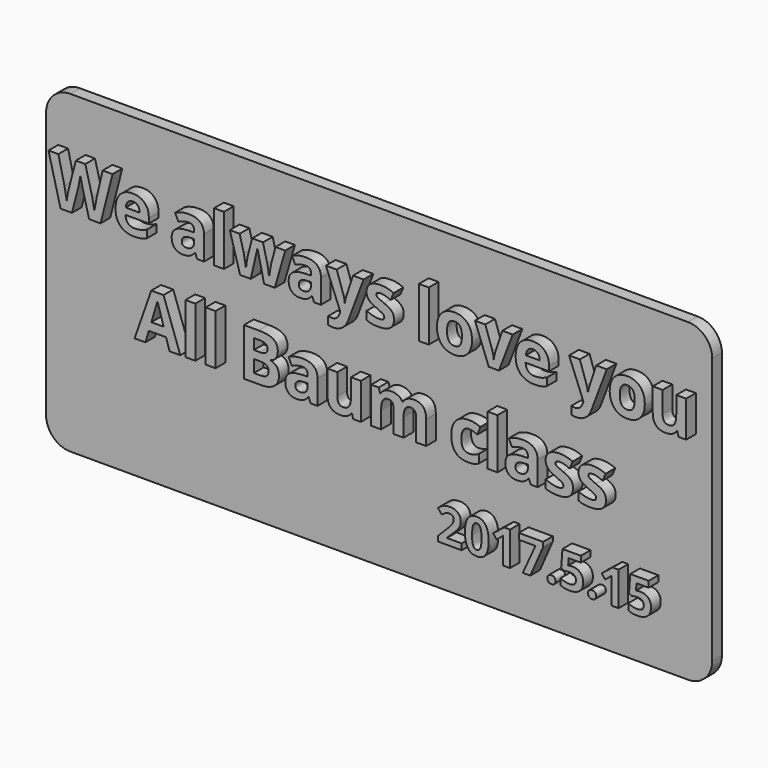
from build123d import *

# Parameters (mm, degrees)
F0_W           = 55
F0_H           = 26
F1_DEPTH       = 1
F2_TEXT_SIZE   = 5.4704383447
F2_TEXT_SIZE_2 = 3.9251763263
F3_DEPTH       = 1
F4_R           = 2


# Not quite as in the source:
# - Text() gives the source's letters only with a copy of the font that has no kerning and outlines rounded to 1/6400 em; it was checked with that copy


with BuildPart() as f1:
    # F0 (on Front) → F1 (new body)
    with BuildSketch(Plane.XZ):
        Rectangle(F0_W, F0_H)
    extrude(amount=F1_DEPTH)

    # F2 (on face) → F3 (join)
    with BuildSketch(Plane.XZ.offset(1)):
        with Locations((-26.5, 5.0612843918)):
            Text('We always love you', F2_TEXT_SIZE, font='Open Sans', font_style=FontStyle.BOLD, text_align=(TextAlign.LEFT, TextAlign.BOTTOM))
        with Locations((-19.3927039319, -2.3785117569)):
            Text('All Baum class', F2_TEXT_SIZE, font='Open Sans', font_style=FontStyle.BOLD, text_align=(TextAlign.LEFT, TextAlign.BOTTOM))
        with Locations((5.5, -9)):
            Text('2017.5.15', F2_TEXT_SIZE_2, font='Open Sans', font_style=FontStyle.BOLD, text_align=(TextAlign.LEFT, TextAlign.BOTTOM))
    extrude(amount=F3_DEPTH)

    # F4
    f4_edges = [f1.edges().sort_by_distance(p)[0] for p in [
        (-27.5, -0.5, 13),
        (-27.5, -0.5, -13),
        (27.5, -0.5, 13),
        (27.5, -0.5, -13),
    ]]
    fillet(f4_edges, radius=F4_R)


solid = f1.part
